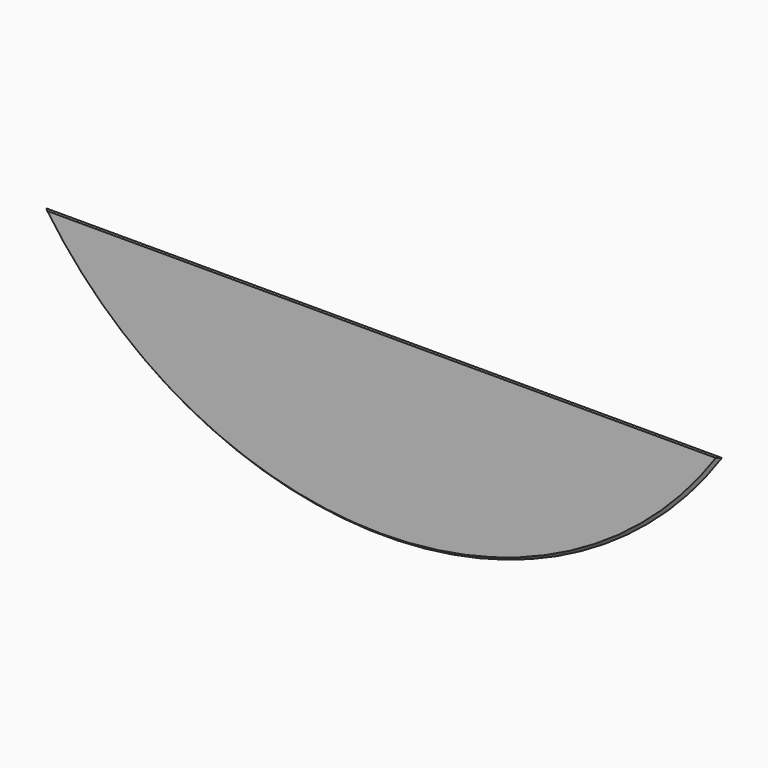
from build123d import *

# Parameters (mm, degrees)
F1_DEPTH    = 1.5
F2_T2_ANGLE = 115.349456206


# Not quite as in the source:
# - a fillet or chamfer that OpenCascade refuses, or shapes differently, is made with other operations: its cross-section is extruded or revolved along the edge and cut away or added


with BuildPart() as f1:
    # F0 (on Front) → F1 (new body, symmetric)
    with BuildSketch(Plane.XZ):
        with BuildLine():
            Line((-244.4200636844, 0), (-339.4112549695, 0))
            ThreePointArc((-339.4112549695, 0), (0, -180), (339.4112549695, 0))
            Line((339.4112549695, 0), (244.4200636844, 0))
            Line((244.4200636844, 0), (254.9738643102, -19.003536996))
            Line((254.9738643102, -19.003536996), (269.4112549695, -45))
            Line((269.4112549695, -45), (239.6748409289, -45))
            Line((239.6748409289, -45), (199.4112549695, -45))
            Line((199.4112549695, -45), (159.1476690102, -45))
            Line((159.1476690102, -45), (129.4112549695, -45))
            Line((129.4112549695, -45), (143.8486452746, -19.0035376339))
            Line((143.8486452746, -19.0035376339), (154.4024462547, 0))
            Line((154.4024462547, 0), (0, 0))
            Line((0, 0), (-154.4024462547, 0))
            Line((-154.4024462547, 0), (-143.8486450184, -19.0035380952))
            Line((-143.8486450184, -19.0035380952), (-129.4112549695, -45))
            Line((-129.4112549695, -45), (-159.1476690102, -45))
            Line((-159.1476690102, -45), (-199.4112549695, -45))
            Line((-199.4112549695, -45), (-239.6748409289, -45))
            Line((-239.6748409289, -45), (-269.4112549695, -45))
            Line((-269.4112549695, -45), (-254.9738639334, -19.0035363174))
            Line((-254.9738639334, -19.0035363174), (-244.4200636844, 0))
        make_face()
        with BuildLine():
            ThreePointArc((-239.6748409289, -45), (-254.7569182799, -36.3758629314), (-254.9738639334, -19.0035363174))
            Line((-254.9738639334, -19.0035363174), (-269.4112549695, -45))
            Line((-269.4112549695, -45), (-239.6748409289, -45))
        make_face()
        with BuildLine():
            Line((-129.4112549695, -45), (-143.8486450184, -19.0035380952))
            ThreePointArc((-143.8486450184, -19.0035380952), (-142.2068467182, -23.1115446827), (-141.6476690102, -27.5))
            ThreePointArc((-141.6476690102, -27.5), (-146.7733003394, -39.8743686708), (-159.1476690102, -45))
            Line((-159.1476690102, -45), (-129.4112549695, -45))
        make_face()
        with BuildLine():
            ThreePointArc((159.1476690102, -45), (144.065592041, -36.3758635803), (143.8486452746, -19.0035376339))
            Line((143.8486452746, -19.0035376339), (129.4112549695, -45))
            Line((129.4112549695, -45), (159.1476690102, -45))
        make_face()
        with BuildLine():
            Line((269.4112549695, -45), (254.9738643102, -19.003536996))
            ThreePointArc((254.9738643102, -19.003536996), (256.6156630632, -23.1115440741), (257.1748409289, -27.5))
            ThreePointArc((257.1748409289, -27.5), (252.0492095997, -39.8743686708), (239.6748409289, -45))
            Line((239.6748409289, -45), (269.4112549695, -45))
        make_face()
        with BuildLine():
            ThreePointArc((176.6476690102, -27.5), (163.5361245829, -10.5591777742), (143.8486452746, -19.0035376339))
            ThreePointArc((143.8486452746, -19.0035376339), (144.065592041, -36.3758635803), (159.1476690102, -45))
            ThreePointArc((159.1476690102, -45), (171.5220376809, -39.8743686708), (176.6476690102, -27.5))
        make_face()
        with BuildLine():
            Line((199.4112549695, -45), (199.4112549695, 0))
            Line((199.4112549695, 0), (154.4024462547, 0))
            Line((154.4024462547, 0), (143.8486452746, -19.0035376339))
            ThreePointArc((143.8486452746, -19.0035376339), (163.5361245829, -10.5591777742), (176.6476690102, -27.5))
            ThreePointArc((176.6476690102, -27.5), (171.5220376809, -39.8743686708), (159.1476690102, -45))
            Line((159.1476690102, -45), (199.4112549695, -45))
        make_face()
        with BuildLine():
            Line((254.9738643102, -19.003536996), (244.4200636844, 0))
            Line((244.4200636844, 0), (199.4112549695, 0))
            Line((199.4112549695, 0), (199.4112549695, -45))
            Line((199.4112549695, -45), (239.6748409289, -45))
            ThreePointArc((239.6748409289, -45), (224.5927637747, -18.6241367341), (254.9738643102, -19.003536996))
        make_face()
        with BuildLine():
            ThreePointArc((257.1748409289, -27.5), (256.6156630632, -23.1115440741), (254.9738643102, -19.003536996))
            ThreePointArc((254.9738643102, -19.003536996), (224.5927637747, -18.6241367341), (239.6748409289, -45))
            ThreePointArc((239.6748409289, -45), (252.0492095997, -39.8743686708), (257.1748409289, -27.5))
        make_face()
        with BuildLine():
            ThreePointArc((-222.1748409289, -27.5), (-235.2863846273, -10.559177963), (-254.9738639334, -19.0035363174))
            ThreePointArc((-254.9738639334, -19.0035363174), (-254.7569182799, -36.3758629314), (-239.6748409289, -45))
            ThreePointArc((-239.6748409289, -45), (-227.3004722581, -39.8743686708), (-222.1748409289, -27.5))
        make_face()
        with BuildLine():
            Line((-199.4112549695, 0), (-244.4200636844, 0))
            Line((-244.4200636844, 0), (-254.9738639334, -19.0035363174))
            ThreePointArc((-254.9738639334, -19.0035363174), (-235.2863846273, -10.559177963), (-222.1748409289, -27.5))
            ThreePointArc((-222.1748409289, -27.5), (-227.3004722581, -39.8743686708), (-239.6748409289, -45))
            Line((-239.6748409289, -45), (-199.4112549695, -45))
            Line((-199.4112549695, -45), (-199.4112549695, 0))
        make_face()
        with BuildLine():
            Line((-154.4024462547, 0), (-199.4112549695, 0))
            Line((-199.4112549695, 0), (-199.4112549695, -45))
            Line((-199.4112549695, -45), (-159.1476690102, -45))
            ThreePointArc((-159.1476690102, -45), (-174.2297458455, -18.6241361923), (-143.8486450184, -19.0035380952))
            Line((-143.8486450184, -19.0035380952), (-154.4024462547, 0))
        make_face()
        with BuildLine():
            ThreePointArc((-141.6476690102, -27.5), (-142.2068467182, -23.1115446827), (-143.8486450184, -19.0035380952))
            ThreePointArc((-143.8486450184, -19.0035380952), (-174.2297458455, -18.6241361923), (-159.1476690102, -45))
            ThreePointArc((-159.1476690102, -45), (-146.7733003394, -39.8743686708), (-141.6476690102, -27.5))
        make_face()
    extrude(amount=F1_DEPTH, both=True)

    # F2: chamfer of 5 on 1 edges, made by hand

    # F2_s1 → F2_t2 (revolve, cut)
    with BuildSketch(Plane(origin=(-103.9270328196, 0, 164.2358796947), x_dir=(0, 1, 0), z_dir=(-0.5347251236, 0, 0.84502606))):
        Polygon((3.5, 287.0132215633), (-1.5, 282.0132215633), (-1.5, 287.0132215633), align=None)
    revolve(axis=Axis((0, -1.5, 230), (0, -1, 0)), revolution_arc=F2_T2_ANGLE, mode=Mode.SUBTRACT)


solid = f1.part
